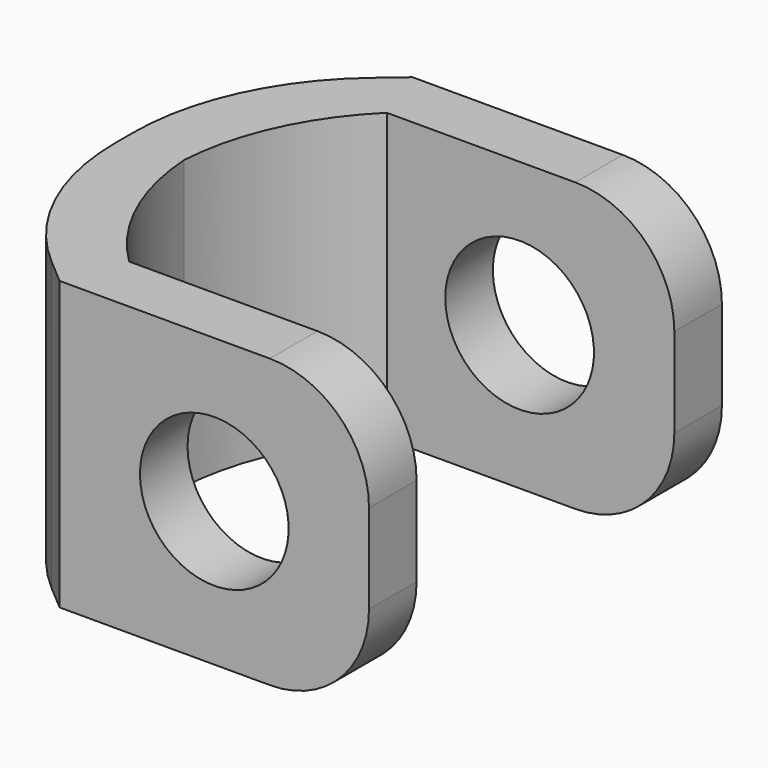
from build123d import *

# Parameters (mm, degrees)
F2_DEPTH    = 5.8
F3_T1_DEPTH = 17.3214031257
F3_T3_DEPTH = 5.8
F5_DEPTH    = 8.901
F6_R        = 2


# Not quite as in the source:
# - a fillet or chamfer that OpenCascade refuses, or shapes differently, is made with other operations: its cross-section is extruded or revolved along the edge and cut away or added


with BuildPart() as f2:
    # F1 (on Top) → F2 (new body)
    with BuildSketch(Plane.XY):
        Polygon((-7.2977824063, -1.970131098), (-7.2977824063, 0), (-7.2977824063, 1.970131098), (-5.8, 3.25), (0, 3.25), (0, 4.45), (-6.2428722575, 4.45), (-8.4977824063, 2.523158448), (-8.4977824063, 0), (-8.4977824063, -2.523158448), (-6.2428722575, -4.45), (0, -4.45), (0, -3.25), (-5.8, -3.25), align=None)
    extrude(amount=F2_DEPTH)

    # F3: fillet of radius 5 on 4 edges, made by hand

    # F3_s2 → F3_t1 (cut)
    with BuildSketch(Plane.XY.offset(-5.7607015629)):
        with BuildLine():
            ThreePointArc((-6.7459644775, -4.0201030507), (-8.0387575415, -2.3116140275), (-8.4977824063, -0.2188778229))
            Line((-8.4977824063, -0.2188778229), (-8.5977824063, -0.2188778229))
            Line((-8.5977824063, -0.2188778229), (-8.5977824063, -2.5692440605))
            Line((-8.5977824063, -2.5692440605), (-6.8109281189, -4.0961275552))
            Line((-6.8109281189, -4.0961275552), (-6.7459644775, -4.0201030507))
        make_face()
        with BuildLine():
            ThreePointArc((-8.4977824063, 0.2188778229), (-8.0387575415, 2.3116140275), (-6.7459644775, 4.0201030507))
            Line((-6.7459644775, 4.0201030507), (-6.8109281189, 4.0961275552))
            Line((-6.8109281189, 4.0961275552), (-8.5977824063, 2.5692440605))
            Line((-8.5977824063, 2.5692440605), (-8.5977824063, 0.2188778229))
            Line((-8.5977824063, 0.2188778229), (-8.4977824063, 0.2188778229))
        make_face()
    extrude(amount=F3_T1_DEPTH, mode=Mode.SUBTRACT)

    # F3_s4 → F3_t3 (join)
    with BuildSketch(Plane.XY):
        with BuildLine():
            ThreePointArc((-7.2977824063, 0.3185391867), (-6.9081559253, -1.6165205064), (-5.8, -3.25))
            Line((-5.8, -3.25), (-5.8700443519, -3.3213707837))
            ThreePointArc((-5.8700443519, -3.3213707837), (-6.6138548446, -2.6860900535), (-7.3627460478, -2.0461556025))
            Line((-7.3627460478, -2.0461556025), (-7.3977824063, -1.970131098))
            Line((-7.3977824063, -1.970131098), (-7.3977824063, 0.3185391867))
            Line((-7.3977824063, 0.3185391867), (-7.2977824063, 0.3185391867))
        make_face()
        with BuildLine():
            ThreePointArc((-7.2977824063, -0.3185391867), (-6.9081559253, 1.6165205064), (-5.8, 3.25))
            Line((-5.8, 3.25), (-5.8700443519, 3.3213707837))
            ThreePointArc((-5.8700443519, 3.3213707837), (-6.6138548446, 2.6860900535), (-7.3627460478, 2.0461556025))
            Line((-7.3627460478, 2.0461556025), (-7.3977824063, 1.970131098))
            Line((-7.3977824063, 1.970131098), (-7.3977824063, -0.3185391867))
            Line((-7.3977824063, -0.3185391867), (-7.2977824063, -0.3185391867))
        make_face()
    extrude(amount=F3_T3_DEPTH)

    # F4 (on face) → F5 (cut, through all)
    with BuildSketch(Plane.XZ.offset(4.45)):
        with BuildLine():
            Line((-4.6214361287, 2.9), (-3.1214361287, 2.9))
            Line((-3.1214361287, 2.9), (-1.6214361287, 2.9))
            ThreePointArc((-1.6214361287, 2.9), (-3.1214361287, 4.4), (-4.6214361287, 2.9))
        make_face()
        with BuildLine():
            Line((-1.6214361287, 2.9), (-3.1214361287, 2.9))
            Line((-3.1214361287, 2.9), (-4.6214361287, 2.9))
            ThreePointArc((-4.6214361287, 2.9), (-3.1214361287, 1.4), (-1.6214361287, 2.9))
        make_face()
    extrude(amount=-F5_DEPTH, mode=Mode.SUBTRACT)

    # F6
    f6_edges = [f2.edges().sort_by_distance(p)[0] for p in [
        (0, 3.85, 5.8),
        (0, -3.85, 5.8),
        (0, 3.85, 0),
        (0, -3.85, 0),
    ]]
    fillet(f6_edges, radius=F6_R)


solid = f2.part
